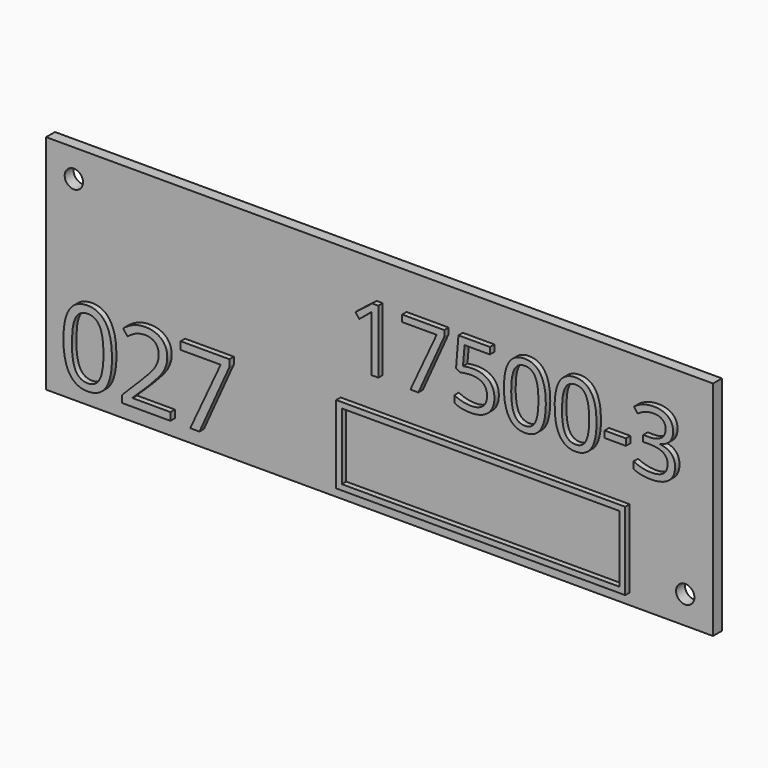
from build123d import *

# Parameters (mm, degrees)
F0_W         = 120
F0_H         = 40
F1_DEPTH     = 2
F3_D         = 3.3
F4_TEXT_SIZE = 15.9647445225
F5_DEPTH     = 1
F6_TEXT_SIZE = 18.5054667028
F7_DEPTH     = 1
F8_W         = 52
F8_H         = 14
F8_W_2       = 49.99999962
F8_H_2       = 11.99999962
F9_DEPTH     = 1


# Not quite as in the source:
# - Text() gives the source's letters only with a copy of the font that has no kerning and outlines rounded to 1/6400 em; it was checked with that copy


with BuildPart() as f1:
    # F0 (on Front) → F1 (new body)
    with BuildSketch(Plane.XZ):
        Rectangle(F0_W, F0_H)
    extrude(amount=F1_DEPTH)

    # F3 (through all)
    with Locations(Plane.XZ.offset(2)):
        with Locations((-55, 15), (55, -15)):
            Hole(F3_D / 2)

    # F4 (on face) → F5 (join)
    with BuildSketch(Plane.XZ.offset(2)):
        with Locations((-5, 2)):
            Text('17500-3', F4_TEXT_SIZE, font='Open Sans', text_align=(TextAlign.LEFT, TextAlign.BOTTOM))
    extrude(amount=F5_DEPTH)

    # F6 (on face) → F7 (join)
    with BuildSketch(Plane.XZ.offset(2)):
        with Locations((-57, -17)):
            Text('027', F6_TEXT_SIZE, font='Open Sans', text_align=(TextAlign.LEFT, TextAlign.BOTTOM))
    extrude(amount=F7_DEPTH)

    # F8 (on face) → F9 (join)
    with BuildSketch(Plane.XZ.offset(2)):
        with Locations((19, -11)):
            Rectangle(F8_W, F8_H)
        with Locations((19, -11)):
            Rectangle(F8_W_2, F8_H_2, mode=Mode.SUBTRACT)
    extrude(amount=F9_DEPTH)


solid = f1.part
